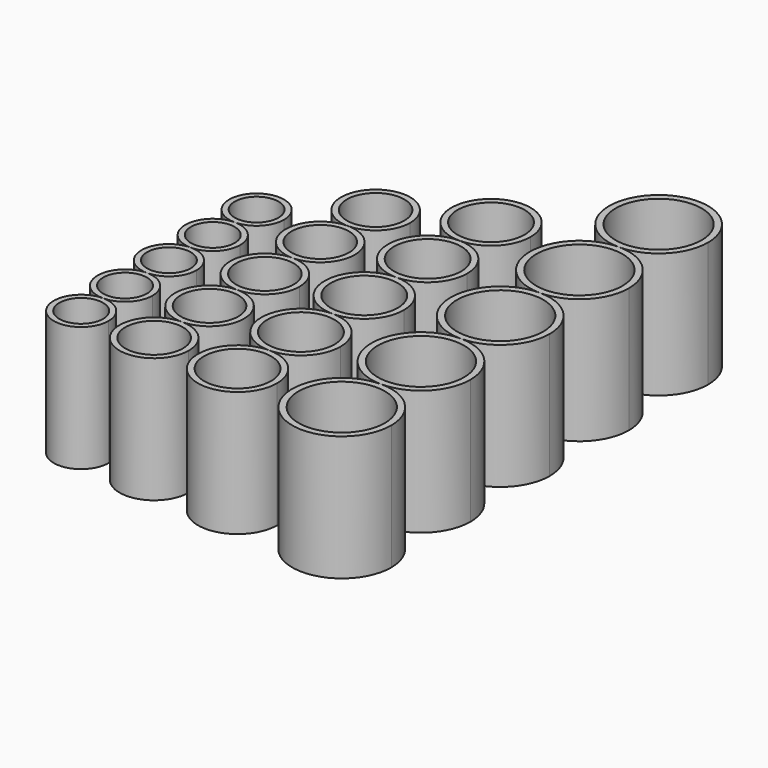
from build123d import *

# Parameters (mm, degrees)
F5_R     = 20.447
F6_DEPTH = 76.2
F5_R_2   = 26.2509
F5_R_3   = 17.526
F5_R_4   = 13.3223


# Not quite as in the source:
# - a variable given as a bare number and used for a length is read in inches; the dataset says mm whatever the document's units were
# - the program builds the solid bodies; features that only make, move or delete a surface that nothing else refers to are left out


with BuildPart() as f6:
    # F5 (on Top) → F6 (new body)
    with BuildSketch(Plane.XY):
        with BuildLine():
            ThreePointArc((2.415e-07, 24.13), (-17.0624867154, -17.0624865447), (24.13, 0))
            ThreePointArc((24.13, 0), (17.0624867154, 17.0624865447), (2.415e-07, 24.13))
        make_face()
        Circle(F5_R, mode=Mode.SUBTRACT)
    extrude(amount=F6_DEPTH)


with BuildPart() as f6b:
    # F5 (on Top) → F6, piece 2 (new body)
    with BuildSketch(Plane.XY):
        with BuildLine():
            ThreePointArc((24.13, 193.04), (-17.0624866044, 210.1024866557), (-7.25e-08, 168.91))
            ThreePointArc((-7.25e-08, 168.91), (17.0624866044, 175.9775133443), (24.13, 193.04))
        make_face()
        with Locations((0, 193.04)):
            Circle(F5_R, mode=Mode.SUBTRACT)
    extrude(amount=F6_DEPTH)


with BuildPart() as f6c:
    # F5 (on Top) → F6, piece 3 (new body)
    with BuildSketch(Plane.XY):
        with BuildLine():
            ThreePointArc((-7.25e-08, 168.91), (-24.13, 144.7800000021), (-7.68e-08, 120.65))
            ThreePointArc((-7.68e-08, 120.65), (17.0624866029, 127.7175133428), (24.13, 144.78))
            ThreePointArc((24.13, 144.78), (17.0624866044, 161.8424866557), (-7.25e-08, 168.91))
        make_face()
        with Locations((0, 144.78)):
            Circle(F5_R, mode=Mode.SUBTRACT)
    extrude(amount=F6_DEPTH)


with BuildPart() as f6d:
    # F5 (on Top) → F6, piece 4 (new body)
    with BuildSketch(Plane.XY):
        with BuildLine():
            ThreePointArc((-7.68e-08, 120.65), (-24.13, 96.5200000237), (-1.242e-07, 72.39))
            ThreePointArc((-1.242e-07, 72.39), (17.0624865861, 79.4575133261), (24.13, 96.52))
            ThreePointArc((24.13, 96.52), (17.0624866029, 113.5824866572), (-7.68e-08, 120.65))
        make_face()
        with Locations((0, 96.52)):
            Circle(F5_R, mode=Mode.SUBTRACT)
    extrude(amount=F6_DEPTH)


with BuildPart() as f6e:
    # F5 (on Top) → F6, piece 5 (new body)
    with BuildSketch(Plane.XY):
        with BuildLine():
            ThreePointArc((-1.242e-07, 72.39), (-24.13, 48.2599998172), (2.415e-07, 24.13))
            ThreePointArc((2.415e-07, 24.13), (17.0624867154, 31.1975134553), (24.13, 48.26))
            ThreePointArc((24.13, 48.26), (17.0624865861, 65.3224866739), (-1.242e-07, 72.39))
        make_face()
        with Locations((0, 48.26)):
            Circle(F5_R, mode=Mode.SUBTRACT)
    extrude(amount=F6_DEPTH)


with BuildPart() as f6f:
    # F5 (on Top) → F6, piece 6 (new body)
    with BuildSketch(Plane.XY):
        with BuildLine():
            ThreePointArc((63.5, 30.1625), (42.1718917125, -21.3281082875), (93.6625, 0))
            ThreePointArc((93.6625, 0), (84.8281082875, 21.3281082875), (63.5, 30.1625))
        make_face()
        with Locations((63.5, 0)):
            Circle(F5_R_2, mode=Mode.SUBTRACT)
    extrude(amount=F6_DEPTH)


with BuildPart() as f6g:
    # F5 (on Top) → F6, piece 7 (new body)
    with BuildSketch(Plane.XY):
        with BuildLine():
            ThreePointArc((93.6625, 241.3), (42.1718916511, 262.6281082262), (63.5000001735, 211.1375))
            ThreePointArc((63.5000001735, 211.1375), (84.8281083489, 219.9718917738), (93.6625, 241.3))
        make_face()
        with Locations((63.5, 241.3)):
            Circle(F5_R_2, mode=Mode.SUBTRACT)
    extrude(amount=F6_DEPTH)


with BuildPart() as f6h:
    # F5 (on Top) → F6, piece 8 (new body)
    with BuildSketch(Plane.XY):
        with BuildLine():
            ThreePointArc((63.5000001735, 211.1375), (33.3375, 180.9750000105), (63.5000001525, 150.8125))
            ThreePointArc((63.5000001525, 150.8125), (84.8281083415, 159.6468917664), (93.6625, 180.975))
            ThreePointArc((93.6625, 180.975), (84.8281083489, 202.3031082262), (63.5000001735, 211.1375))
        make_face()
        with Locations((63.5, 180.975)):
            Circle(F5_R_2, mode=Mode.SUBTRACT)
    extrude(amount=F6_DEPTH)


with BuildPart() as f6i:
    # F5 (on Top) → F6, piece 9 (new body)
    with BuildSketch(Plane.XY):
        with BuildLine():
            ThreePointArc((63.5000001525, 150.8125), (33.3375, 120.6500000068), (63.5000001389, 90.4875))
            ThreePointArc((63.5000001389, 90.4875), (84.8281083366, 99.3218917616), (93.6625, 120.65))
            ThreePointArc((93.6625, 120.65), (84.8281083415, 141.9781082336), (63.5000001525, 150.8125))
        make_face()
        with Locations((63.5, 120.65)):
            Circle(F5_R_2, mode=Mode.SUBTRACT)
    extrude(amount=F6_DEPTH)


with BuildPart() as f6j:
    # F5 (on Top) → F6, piece 10 (new body)
    with BuildSketch(Plane.XY):
        with BuildLine():
            ThreePointArc((63.5000001389, 90.4875), (33.3375, 60.3250000694), (63.5, 30.1625))
            ThreePointArc((63.5, 30.1625), (84.8281082875, 38.9968917125), (93.6625, 60.325))
            ThreePointArc((93.6625, 60.325), (84.8281083366, 81.6531082384), (63.5000001389, 90.4875))
        make_face()
        with Locations((63.5, 60.325)):
            Circle(F5_R_2, mode=Mode.SUBTRACT)
    extrude(amount=F6_DEPTH)


with BuildPart() as f6k:
    # F5 (on Top) → F6, piece 11 (new body)
    with BuildSketch(Plane.XY):
        with BuildLine():
            ThreePointArc((-50.8, 21.082), (-65.707225161, -14.907225161), (-29.718, 0))
            ThreePointArc((-29.718, 0), (-35.892774839, 14.907225161), (-50.8, 21.082))
        make_face()
        with Locations((-50.8, 0)):
            Circle(F5_R_3, mode=Mode.SUBTRACT)
    extrude(amount=F6_DEPTH)


with BuildPart() as f6l:
    # F5 (on Top) → F6, piece 12 (new body)
    with BuildSketch(Plane.XY):
        with BuildLine():
            ThreePointArc((-29.718, 168.656), (-65.707225161, 183.563225161), (-50.8, 147.574))
            ThreePointArc((-50.8, 147.574), (-35.892774839, 153.748774839), (-29.718, 168.656))
        make_face()
        with Locations((-50.8, 168.656)):
            Circle(F5_R_3, mode=Mode.SUBTRACT)
    extrude(amount=F6_DEPTH)


with BuildPart() as f6m:
    # F5 (on Top) → F6, piece 13 (new body)
    with BuildSketch(Plane.XY):
        with BuildLine():
            ThreePointArc((-50.8, 147.574), (-71.882, 126.4919999282), (-50.7999998565, 105.41))
            ThreePointArc((-50.7999998565, 105.41), (-35.8927747883, 111.5847748898), (-29.718, 126.492))
            ThreePointArc((-29.718, 126.492), (-35.892774839, 141.399225161), (-50.8, 147.574))
        make_face()
        with Locations((-50.8, 126.492)):
            Circle(F5_R_3, mode=Mode.SUBTRACT)
    extrude(amount=F6_DEPTH)


with BuildPart() as f6n:
    # F5 (on Top) → F6, piece 14 (new body)
    with BuildSketch(Plane.XY):
        with BuildLine():
            ThreePointArc((-50.7999998565, 105.41), (-71.882, 84.3280001019), (-50.8000000603, 63.246))
            ThreePointArc((-50.8000000603, 63.246), (-35.8927748604, 69.4207748177), (-29.718, 84.328))
            ThreePointArc((-29.718, 84.328), (-35.8927747883, 99.2352251102), (-50.7999998565, 105.41))
        make_face()
        with Locations((-50.8, 84.328)):
            Circle(F5_R_3, mode=Mode.SUBTRACT)
    extrude(amount=F6_DEPTH)


with BuildPart() as f6o:
    # F5 (on Top) → F6, piece 15 (new body)
    with BuildSketch(Plane.XY):
        with BuildLine():
            ThreePointArc((-50.8000000603, 63.246), (-71.882, 42.1639999698), (-50.8, 21.082))
            ThreePointArc((-50.8, 21.082), (-35.892774839, 27.256774839), (-29.718, 42.164))
            ThreePointArc((-29.718, 42.164), (-35.8927748604, 57.0712251823), (-50.8000000603, 63.246))
        make_face()
        with Locations((-50.8, 42.164)):
            Circle(F5_R_3, mode=Mode.SUBTRACT)
    extrude(amount=F6_DEPTH)


with BuildPart() as f6p:
    # F5 (on Top) → F6, piece 16 (new body)
    with BuildSketch(Plane.XY):
        with BuildLine():
            ThreePointArc((-95.25, 16.7005), (-107.0590367992, -11.8090367992), (-78.5495, 0))
            ThreePointArc((-78.5495, 0), (-83.4409632008, 11.8090367992), (-95.25, 16.7005))
        make_face()
        with Locations((-95.25, 0)):
            Circle(F5_R_4, mode=Mode.SUBTRACT)
    extrude(amount=F6_DEPTH)


with BuildPart() as f6q:
    # F5 (on Top) → F6, piece 17 (new body)
    with BuildSketch(Plane.XY):
        with BuildLine():
            ThreePointArc((-78.5495, 133.604), (-107.0590367992, 145.4130367992), (-95.25, 116.9035))
            ThreePointArc((-95.25, 116.9035), (-83.4409632008, 121.7949632008), (-78.5495, 133.604))
        make_face()
        with Locations((-95.25, 133.604)):
            Circle(F5_R_4, mode=Mode.SUBTRACT)
    extrude(amount=F6_DEPTH)


with BuildPart() as f6r:
    # F5 (on Top) → F6, piece 18 (new body)
    with BuildSketch(Plane.XY):
        with BuildLine():
            ThreePointArc((-95.25, 116.9035), (-111.9505, 100.203), (-95.25, 83.5025))
            ThreePointArc((-95.25, 83.5025), (-83.4409632008, 88.3939632008), (-78.5495, 100.203))
            ThreePointArc((-78.5495, 100.203), (-83.4409632008, 112.0120367992), (-95.25, 116.9035))
        make_face()
        with Locations((-95.25, 100.203)):
            Circle(F5_R_4, mode=Mode.SUBTRACT)
    extrude(amount=F6_DEPTH)


with BuildPart() as f6s:
    # F5 (on Top) → F6, piece 19 (new body)
    with BuildSketch(Plane.XY):
        with BuildLine():
            ThreePointArc((-95.25, 83.5025), (-111.9505, 66.802), (-95.25, 50.1015))
            ThreePointArc((-95.25, 50.1015), (-83.4409632008, 54.9929632008), (-78.5495, 66.802))
            ThreePointArc((-78.5495, 66.802), (-83.4409632008, 78.6110367992), (-95.25, 83.5025))
        make_face()
        with Locations((-95.25, 66.802)):
            Circle(F5_R_4, mode=Mode.SUBTRACT)
    extrude(amount=F6_DEPTH)


with BuildPart() as f6t:
    # F5 (on Top) → F6, piece 20 (new body)
    with BuildSketch(Plane.XY):
        with BuildLine():
            ThreePointArc((-95.25, 50.1015), (-111.9505, 33.401), (-95.25, 16.7005))
            ThreePointArc((-95.25, 16.7005), (-83.4409632008, 21.5919632008), (-78.5495, 33.401))
            ThreePointArc((-78.5495, 33.401), (-83.4409632008, 45.2100367992), (-95.25, 50.1015))
        make_face()
        with Locations((-95.25, 33.401)):
            Circle(F5_R_4, mode=Mode.SUBTRACT)
    extrude(amount=F6_DEPTH)


solid = Compound([f6.part, f6b.part, f6c.part, f6d.part, f6e.part, f6f.part, f6g.part, f6h.part, f6i.part, f6j.part, f6k.part, f6l.part, f6m.part, f6n.part, f6o.part, f6p.part, f6q.part, f6r.part, f6s.part, f6t.part])
